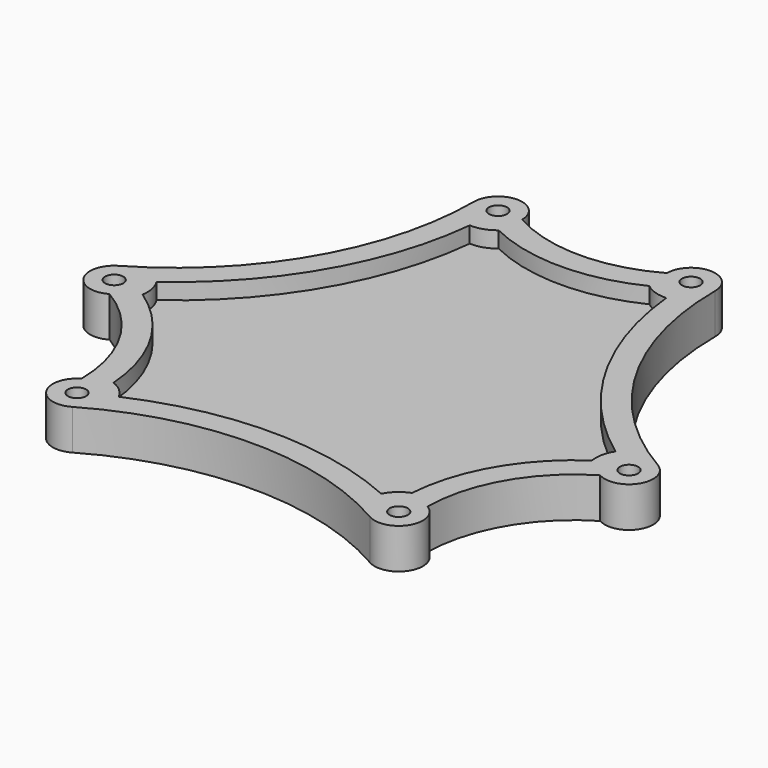
from build123d import *

# Parameters (mm, degrees)
F2_DEPTH    = 5
F3_D        = 2.2606
F4_T        = 3
F4_T3_DEPTH = 11


# Not quite as in the source:
# - a shell that OpenCascade refuses in one call is made with other operations: the cavity is built on its own and cut out


with BuildPart() as f2:
    # F1 (on Top) → F2 (new body)
    with BuildSketch(Plane.XY):
        with BuildLine():
            ThreePointArc((9, 30.0222139979), (0, 27.6692232402), (-9, 30.0222139979))
            ThreePointArc((-9, 30.0222139979), (-12, 33.0222139979), (-15, 30.0222139979))
            ThreePointArc((-15, 30.0222139979), (-19.95706006, 11.5222139979), (-33.5, -2.0207259422))
            ThreePointArc((-33.5, -2.0207259422), (-34.5980762114, -6.1188021535), (-30.5, -7.2168783649))
            ThreePointArc((-30.5, -7.2168783649), (-23.962250229, -13.8346116201), (-21.5, -22.805335633))
            ThreePointArc((-21.5, -22.805335633), (-22.5980762114, -26.9034118443), (-18.5, -28.0014880557))
            ThreePointArc((-18.5, -28.0014880557), (0, -23.0444279957), (18.5, -28.0014880557))
            ThreePointArc((18.5, -28.0014880557), (22.5980762114, -26.9034118443), (21.5, -22.805335633))
            ThreePointArc((21.5, -22.805335633), (23.962250229, -13.8346116201), (30.5, -7.2168783649))
            ThreePointArc((30.5, -7.2168783649), (34.5980762114, -6.1188021535), (33.5, -2.0207259422))
            ThreePointArc((33.5, -2.0207259422), (19.95706006, 11.5222139979), (15, 30.0222139979))
            ThreePointArc((15, 30.0222139979), (12, 33.0222139979), (9, 30.0222139979))
        make_face()
    extrude(amount=F2_DEPTH)

    # F3 (through all)
    with Locations(Plane(origin=(0, 0, 0), x_dir=(1, 0, 0), z_dir=(0, 0, -1))):
        with Locations((-12, -30.0222139979), (12, -30.0222139979), (32, 4.6188021535), (20, 25.4034118443), (-20, 25.4034118443), (-32, 4.6188021535)):
            Hole(F3_D / 2)

    # F4: shell of thickness 3, made by hand


with BuildPart() as f4_core1:
    # F4_t2: copy of F2
    add(f2.part)

    # the walls: a layer under each face that stays
    f4_faces = [f4_core1.faces().sort_by_distance(p)[0] for p in [
        (0, -23.0444279957, 2.5),
        (0, 2.3094010768, 0),
        (-23.962250229, -13.8346116201, 2.5),
        (23.962250229, -13.8346116201, 2.5),
        (-19.95706006, 11.5222139979, 2.5),
        (19.95706006, 11.5222139979, 2.5),
        (0, 27.6692232402, 2.5),
        (-21.1303, -25.4034118443, 2.5),
        (-33.1303, -4.6188021535, 2.5),
        (18.8697, -25.4034118443, 2.5),
        (30.8697, -4.6188021535, 2.5),
        (-13.1303, 30.0222139979, 2.5),
        (10.8697, 30.0222139979, 2.5),
    ]]
    thicken(f4_faces, amount=-F4_T, mode=Mode.SUBTRACT)

    # F4_s4 → F4_t3 (cut)
    with BuildSketch(Plane.XY.offset(-3)):
        Polygon((-21.5449977822, -22.7797196489), (-20, -25.4034118443), (-18.4788645602, -24.5251838887), (-18.5002217799, -22.7688578263), align=None)
        Polygon((21.5449977822, -22.7797196489), (20, -25.4034118443), (18.4788645602, -24.5251838887), (18.5002217799, -22.7688578263), align=None)
        Polygon((-30.5003147982, -7.2686555794), (-28.9685201827, -4.6372331239), (-30.4788645602, -3.7405741979), (-32, -4.6188021535), align=None)
        Polygon((30.5003147982, -7.2686555794), (28.9685201827, -4.6372331239), (30.4788645602, -3.7405741979), (32, -4.6188021535), align=None)
        Polygon((-8.955317016, 30.0483752283), (-12, 30.0222139979), (-12, 28.2657580866), (-10.4682984028, 27.4060909502), align=None)
        Polygon((8.955317016, 30.0483752283), (12, 30.0222139979), (12, 28.2657580866), (10.4682984028, 27.4060909502), align=None)
    extrude(amount=F4_T3_DEPTH, mode=Mode.SUBTRACT)


with BuildPart() as f2_1:
    add(f2.part)

    # what is left inside the walls is the cavity
    f4_cavity = [f4_core1.part.solids().sort_by_distance(p)[0] for p in [
        (0, -6.739348, 4.97),
    ]]
    add(f4_cavity, mode=Mode.SUBTRACT)


solid = f2_1.part
